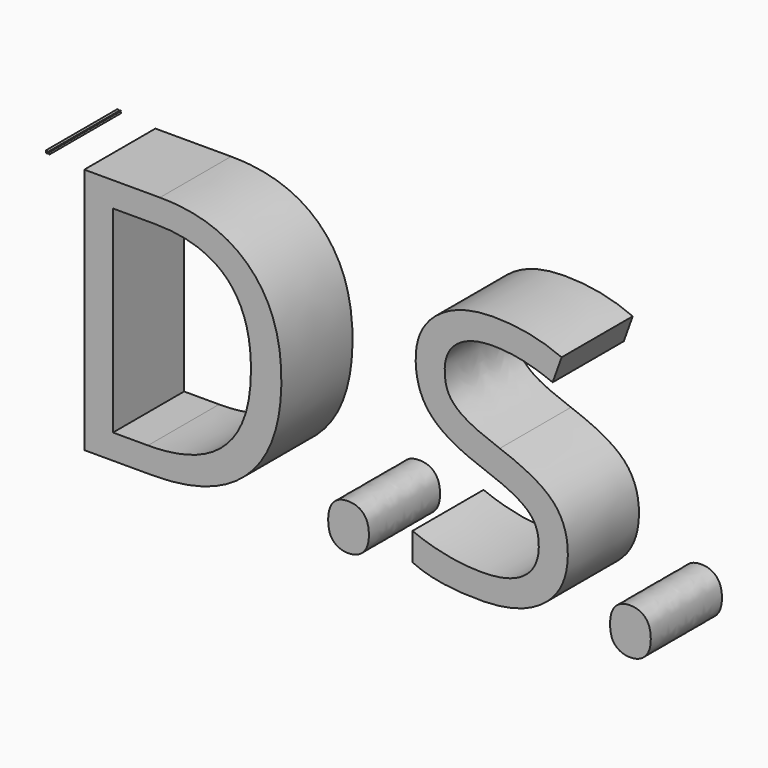
from build123d import *

# Parameters (mm, degrees)
F0_TEXT_SIZE   = 1.0154184161
F0_TEXT_SIZE_2 = 98.8031659896
F1_DEPTH       = 25.4


# Not quite as in the source:
# - Text() gives the source's letters only with a copy of the font that has no kerning and outlines rounded to 1/6400 em; it was checked with that copy


with BuildPart() as f1:
    # F0 (on Front) → F1 (new body)
    with BuildSketch(Plane.XZ):
        with Locations((-71.7116519809, 21.8676049262)):
            Text('DS', F0_TEXT_SIZE, font='Open Sans', text_align=(TextAlign.LEFT, TextAlign.BOTTOM))
        with Locations((-70.3968437912, -49.2706745863)):
            Text('D.S.', F0_TEXT_SIZE_2, font='Open Sans', text_align=(TextAlign.LEFT, TextAlign.BOTTOM))
    extrude(amount=F1_DEPTH)


solid = f1.part
